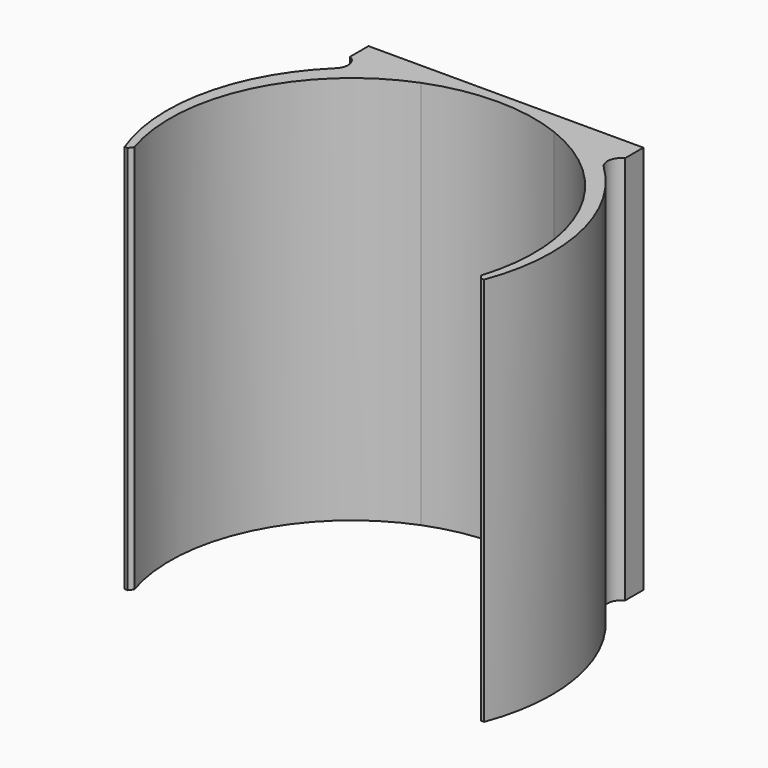
from build123d import *

# Parameters (mm, degrees)
F0_W        = 60
F0_H        = 85
F1_DEPTH    = 5
F3_DEPTH    = 85
F4_DEPTH    = 85
F5_T1_DEPTH = 85
F6_T1_DEPTH = 90.0557507085


# Not quite as in the source:
# - a fillet or chamfer that OpenCascade refuses, or shapes differently, is made with other operations: its cross-section is extruded or revolved along the edge and cut away or added


with BuildPart() as f1:
    # F0 (on Front) → F1 (new body)
    with BuildSketch(Plane.XZ):
        Rectangle(F0_W, F0_H)
    extrude(amount=F1_DEPTH)

    # F2 (on face) → F3 (join, through all)
    with BuildSketch(Plane.XY.offset(42.5)):
        with BuildLine():
            Line((-14.5279902258, -5), (-23.2163735325, -5))
            ThreePointArc((-23.2163735325, -5), (-39.9986276925, -27.1894659474), (-39.2300904919, -55))
            Line((-39.2300904919, -55), (-37.5641118623, -55))
            ThreePointArc((-37.5641118623, -55), (-36.1025868185, -25.3667283731), (-14.5279902258, -5))
        make_face()
        with BuildLine():
            Line((23.2163735325, -5), (14.5279902258, -5))
            ThreePointArc((14.5279902258, -5), (36.1025868185, -25.3667283731), (37.5641118623, -55))
            Line((37.5641118623, -55), (39.2300904919, -55))
            ThreePointArc((39.2300904919, -55), (39.9986276925, -27.1894659474), (23.2163735325, -5))
        make_face()
        with BuildLine():
            ThreePointArc((14.5279902258, -5), (0, -2.25), (-14.5279902258, -5))
            Line((-14.5279902258, -5), (14.5279902258, -5))
        make_face()
        with BuildLine():
            Line((14.5279902258, -5), (-14.5279902258, -5))
            ThreePointArc((-14.5279902258, -5), (-36.1025868185, -25.3667283731), (-37.5641118623, -55))
            Line((-37.5641118623, -55), (37.5641118623, -55))
            ThreePointArc((37.5641118623, -55), (36.1025868185, -25.3667283731), (14.5279902258, -5))
        make_face()
    extrude(amount=-F3_DEPTH)

    # F2 (on face) → F4 (cut, through all)
    with BuildSketch(Plane.XY.offset(42.5)):
        with BuildLine():
            Line((14.5279902258, -5), (-14.5279902258, -5))
            ThreePointArc((-14.5279902258, -5), (-36.1025868185, -25.3667283731), (-37.5641118623, -55))
            Line((-37.5641118623, -55), (37.5641118623, -55))
            ThreePointArc((37.5641118623, -55), (36.1025868185, -25.3667283731), (14.5279902258, -5))
        make_face()
        with BuildLine():
            ThreePointArc((14.5279902258, -5), (0, -2.25), (-14.5279902258, -5))
            Line((-14.5279902258, -5), (14.5279902258, -5))
        make_face()
    extrude(amount=-F4_DEPTH, mode=Mode.SUBTRACT)

    # F5: fillet of radius 3 on 2 edges, made by hand

    # F5_s2 → F5_t1 (join)
    with BuildSketch(Plane.XY.offset(-42.5)):
        with BuildLine():
            ThreePointArc((30, -5), (28.3606490054, -7.224664287), (29.2357538945, -9.8458842905))
            ThreePointArc((29.2357538945, -9.8458842905), (26.3377498383, -7.2842097229), (23.2163735325, -5))
            Line((23.2163735325, -5), (30, -5))
        make_face()
        with BuildLine():
            ThreePointArc((-29.2357538945, -9.8458842905), (-28.3606490054, -7.224664287), (-30, -5))
            Line((-30, -5), (-23.2163735325, -5))
            ThreePointArc((-23.2163735325, -5), (-26.3377498383, -7.2842097229), (-29.2357538945, -9.8458842905))
        make_face()
    extrude(amount=F5_T1_DEPTH)

    # F6: chamfer of 1 on 2 edges, made by hand

    # F6_s2 → F6_t1 (cut)
    with BuildSketch(Plane.XY.offset(-45.0278753542)):
        with BuildLine():
            Line((-37.8490587869, -54.0393279007), (-38.5747461473, -55.0322947503))
            Line((-38.5747461473, -55.0322947503), (-38.5747461473, -55.0522947503))
            ThreePointArc((-38.5747461473, -55.0522947503), (-38.0694290048, -55.02), (-37.5641118623, -55.02))
            Line((-37.5641118623, -55.02), (-37.5452116802, -54.9934591195))
            ThreePointArc((-37.5452116802, -54.9934591195), (-37.7059205116, -54.5194432134), (-37.8300033601, -54.0332541283))
            Line((-37.8300033601, -54.0332541283), (-37.8490587869, -54.0393279007))
        make_face()
        with BuildLine():
            Line((38.5747461473, -55.0322947503), (37.8490587869, -54.0393279007))
            Line((37.8490587869, -54.0393279007), (37.8300033601, -54.0332541283))
            ThreePointArc((37.8300033601, -54.0332541283), (37.7059205116, -54.5194432134), (37.5452116802, -54.9934591195))
            Line((37.5452116802, -54.9934591195), (37.5641118623, -55.02))
            ThreePointArc((37.5641118623, -55.02), (38.0694290048, -55.02), (38.5747461473, -55.0522947503))
            Line((38.5747461473, -55.0522947503), (38.5747461473, -55.0322947503))
        make_face()
    extrude(amount=F6_T1_DEPTH, mode=Mode.SUBTRACT)


solid = f1.part
